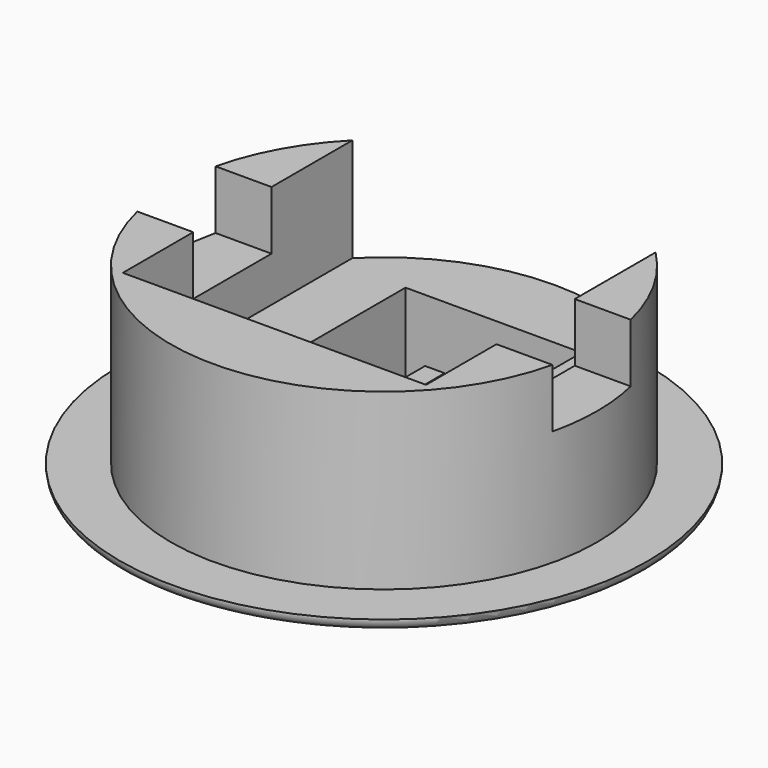
from build123d import *

# Parameters (mm, degrees)
F0_R      = 13.5
F1_DEPTH  = 0.6
F2_R      = 0.59999
F5_R      = 10.9
F6_DEPTH  = 8.9
F9_DEPTH  = 7
F10_DEPTH = 7
F11_DEPTH = 25
F12_DEPTH = 7
F14_DEPTH = 3


# Not quite as in the source:
# - a fillet or chamfer is up to 0.001 mm smaller than in the source, because OpenCascade refuses the exact size


with BuildPart() as f1:
    # F0 (on Top) → F1 (new body)
    with BuildSketch(Plane.XY):
        Circle(F0_R)
    extrude(amount=F1_DEPTH)

    # F2 (radius 0.6 in the source; OpenCascade refuses exactly that, so slightly less here)
    f2_edges = [f1.edges().sort_by_distance(p)[0] for p in [
        (-13.5, 0, 0),
    ]]
    fillet(f2_edges, radius=F2_R)

    # F5 (on face) → F6 (join)
    with BuildSketch(Plane.XY.offset(0.6)):
        Circle(F5_R)
    extrude(amount=F6_DEPTH)

    # F3 (on Front) → F9 (cut)
    with BuildSketch(Plane.XZ):
        Polygon((-0.5, 0), (0, 0), (0.5, 0), (0.5, 1), (1.5, 1), (1.5, 0), (2.5, 0), (2.5, 1), (3.5, 1), (3.5, 0), (4.5, 0), (4.5, 4.2), (-4.5, 4.2), (-4.5, 0), (-3.5, 0), (-3.5, 1), (-2.5, 1), (-2.5, 0), (-1.5, 0), (-1.5, 1), (-0.5, 1), align=None)
    extrude(amount=-F9_DEPTH, mode=Mode.SUBTRACT)

    # F4 (on Front) → F10 (cut)
    with BuildSketch(Plane.XZ):
        Polygon((-0.5, 0), (0, 0), (0.5, 0), (0.5, 1), (1.5, 1), (1.5, 0), (2.5, 0), (2.5, 1), (3.5, 1), (3.5, 0), (4.5, 0), (4.5, 4.2), (-4.5, 4.2), (-4.5, 0), (-3.5, 0), (-3.5, 1), (-2.5, 1), (-2.5, 0), (-1.5, 0), (-1.5, 1), (-0.5, 1), align=None)
    extrude(amount=F10_DEPTH, mode=Mode.SUBTRACT)

    # F7 (on Front) → F11 (cut)
    with BuildSketch(Plane.XZ):
        Polygon((-7.75, 4.2), (0, 4.2), (7.75, 4.2), (7.75, 9.5), (-7.75, 9.5), align=None)
    extrude(amount=-F11_DEPTH, mode=Mode.SUBTRACT)

    # F8 (on Front) → F12 (cut)
    with BuildSketch(Plane.XZ):
        Polygon((-7.75, 4.2), (0, 4.2), (7.75, 4.2), (7.75, 9.5), (-7.75, 9.5), align=None)
    extrude(amount=F12_DEPTH, mode=Mode.SUBTRACT)

    # F13 (on face) → F14 (cut)
    with BuildSketch(Plane.XY.offset(9.5)):
        with BuildLine():
            Line((-7.75, -2.5), (-7.75, 0))
            Line((-7.75, 0), (-7.75, 2.5))
            Line((-7.75, 2.5), (-10.6094297679, 2.5))
            ThreePointArc((-10.6094297679, 2.5), (-10.9, 0), (-10.6094297679, -2.5))
            Line((-10.6094297679, -2.5), (-7.75, -2.5))
        make_face()
        with BuildLine():
            Line((7.75, 2.5), (7.75, 0))
            Line((7.75, 0), (7.75, -2.5))
            Line((7.75, -2.5), (10.6094297679, -2.5))
            ThreePointArc((10.6094297679, -2.5), (10.8271137537, -1.2584147826), (10.9, 0))
            ThreePointArc((10.9, 0), (10.8271137537, 1.2584147826), (10.6094297679, 2.5))
            Line((10.6094297679, 2.5), (7.75, 2.5))
        make_face()
    extrude(amount=-F14_DEPTH, mode=Mode.SUBTRACT)


solid = f1.part
